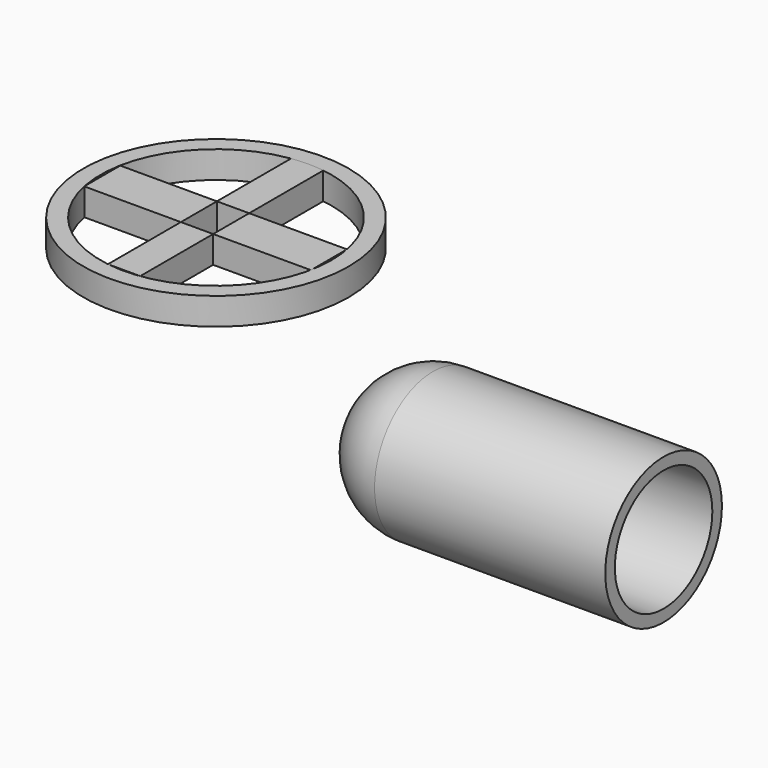
from build123d import *

# Parameters (mm, degrees)
F0_R      = 13.64715261
F1_DEPTH  = 43.18
F4_R      = 11.4040237501
F5_DEPTH  = 43.434
F6_R      = 24.8374772397
F6_R_2    = 21.6302866644
F7_DEPTH  = 12.7
F9_DEPTH  = 5.08
F8_W      = 2.942007035
F8_H      = 17.0599571333
F8_W_2    = 3.09848026
F8_W_3    = 18.0904479147
F8_H_2    = 4.3472547651
F8_H_3    = 4.0815014616
F8_W_4    = 18.2997124576
F10_DEPTH = 7.62


with BuildPart() as f1:
    # F0 (on Right) → F1 (new body)
    with BuildSketch(Plane.YZ):
        Circle(F0_R)
    extrude(amount=F1_DEPTH)

    # F2 (on Top) → F3 (revolve)
    with BuildSketch(Plane.XY):
        with BuildLine():
            Line((0, 0), (0, 13.64715261))
            ThreePointArc((0, 13.64715261), (-9.6499941544, 9.6499941544), (-13.64715261, 0))
            Line((-13.64715261, 0), (0, 0))
        make_face()
    revolve(axis=Axis((-6.823576305, 0, 0), (-1, 0, 0)))

    # F4 (on face) → F5 (cut)
    with BuildSketch(Plane.YZ.offset(43.18)):
        Circle(F4_R)
    extrude(amount=-F5_DEPTH, mode=Mode.SUBTRACT)


with BuildPart() as f7:
    # F6 (on Top) → F7 (new body)
    with BuildSketch(Plane.XY):
        with Locations((-56.3518926501, 19.6899138391)):
            Circle(F6_R)
        with Locations((-56.3518926501, 19.6899138391)):
            Circle(F6_R_2, mode=Mode.SUBTRACT)
    extrude(amount=F7_DEPTH)

    # F10 (cut): a face of the model
    f10_faces = [f7.faces().sort_by_distance(p)[0] for p in [
        (-80.4868599465, 19.6899138391, 0),
    ]]
    extrude(f10_faces, amount=-F10_DEPTH, mode=Mode.SUBTRACT)


with BuildPart() as f9:
    # F8 (on face) → F9 (new body)
    with BuildSketch(Plane.XY.offset(12.7)):
        with BuildLine():
            Line((-59.4503729101, 23.7714153007), (-56.3518926501, 23.7714153007))
            Line((-56.3518926501, 23.7714153007), (-56.3518926501, 41.3202005035))
            ThreePointArc((-56.3518926501, 41.3202005035), (-57.9051426519, 41.2643597327), (-59.4503729101, 41.0971257375))
            Line((-59.4503729101, 41.0971257375), (-59.4503729101, 23.7714153007))
        make_face()
        with BuildLine():
            Line((-56.3518926501, 41.3202005035), (-56.3518926501, 23.7714153007))
            Line((-56.3518926501, 23.7714153007), (-53.4098856151, 23.7714153007))
            Line((-53.4098856151, 23.7714153007), (-53.4098856151, 41.1191904436))
            ThreePointArc((-53.4098856151, 41.1191904436), (-54.8774596711, 41.269889478), (-56.3518926501, 41.3202005035))
        make_face()
    extrude(amount=-F9_DEPTH)


with BuildPart() as f9b:
    # F8 (on face) → F9, piece 2 (new body)
    with BuildSketch(Plane.XY.offset(12.7)):
        with Locations((-54.8808891326, 6.8126805073)):
            Rectangle(F8_W, F8_H)
        with Locations((-57.9011327801, 6.8126805073)):
            Rectangle(F8_W_2, F8_H)
    extrude(amount=-F9_DEPTH)


with BuildPart() as f9c:
    # F8 (on face) → F9, piece 3 (new body)
    with BuildSketch(Plane.XY.offset(12.7)):
        with Locations((-68.4955968675, 17.5162864565)):
            Rectangle(F8_W_3, F8_H_2)
        with Locations((-68.4955968675, 21.7306645699)):
            Rectangle(F8_W_3, F8_H_3)
    extrude(amount=-F9_DEPTH)


with BuildPart() as f9d:
    # F8 (on face) → F9, piece 4 (new body)
    with BuildSketch(Plane.XY.offset(12.7)):
        with Locations((-44.2600293863, 21.7306645699)):
            Rectangle(F8_W_4, F8_H_3)
        with BuildLine():
            Line((-35.1101731575, 19.6899138391), (-53.4098856151, 19.6899138391))
            Line((-53.4098856151, 19.6899138391), (-53.4098856151, 15.342659074))
            Line((-53.4098856151, 15.342659074), (-35.1629644754, 15.342659074))
            ThreePointArc((-35.1629644754, 15.342659074), (-35.1361527014, 15.4754530654), (-35.1101731575, 15.6084123775))
            Line((-35.1101731575, 15.6084123775), (-35.1101731575, 19.6899138391))
        make_face()
    extrude(amount=-F9_DEPTH)


solid = Compound([f1.part, f7.part, f9.part, f9b.part, f9c.part, f9d.part])
